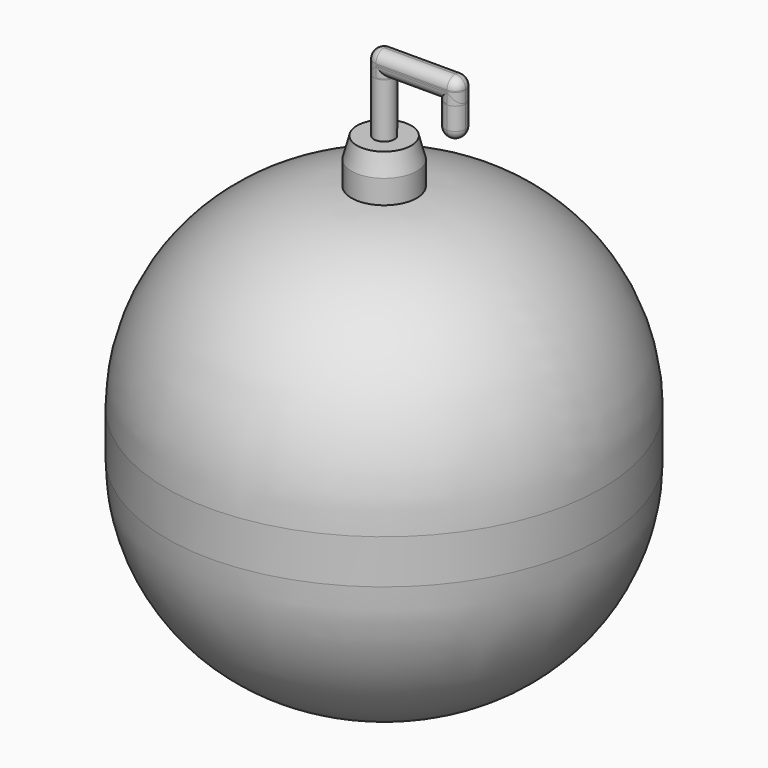
from build123d import *

# Parameters (mm, degrees)
F0_R          = 50
F0_R_2        = 7.5
F1_DEPTH      = 50
F0_R_3        = 2.3544117125
F3_DEPTH      = 50.038
F4_DEPTH      = 50.038
F5_DEPTH      = 10.16
F6_DEPTH      = 25.4
F8_DEPTH      = 2.54
F9_DEPTH      = 10.16
F10_SIZE2     = 4.7397045256
F10_SIZE      = 1.27
F11_R         = 2.286
F12_R         = 2.286
F13_DEPTH     = 2.54
F14_T4_DEPTH  = 27.7630922857
F14_S5_R      = 2.3587376624
F14_T6_DEPTH  = 15
F14_S7_R      = 2.3544117125
F14_T8_DEPTH  = 15
F14_T12_DEPTH = 27.7630922857
F14_S13_R     = 2.3587376624
F14_T14_DEPTH = 15
F14_S15_R     = 2.3544117125
F14_T16_DEPTH = 15


# Not quite as in the source:
# - a fillet or chamfer that OpenCascade refuses, or shapes differently, is made with other operations: its cross-section is extruded or revolved along the edge and cut away or added


with BuildPart() as f1:
    # F0 (on Top) → F1 (new body, symmetric)
    with BuildSketch(Plane.XY):
        Circle(F0_R)
        Circle(F0_R_2, mode=Mode.SUBTRACT)
    extrude(amount=F1_DEPTH, both=True)

    # F2: fillet of radius 45 on 3 edges, made by hand

    # F2_s1 → F2_t2 (revolve, cut)
    with BuildSketch(Plane.XZ):
        with BuildLine():
            ThreePointArc((50, 5.069498111), (37.6917420766, 35.9927903031), (7.5, 50))
            Line((7.5, 50), (50, 50))
            Line((50, 50), (50, 5.069498111))
        make_face()
    revolve(axis=Axis((0, 0, 50), (0, 0, 1)), mode=Mode.SUBTRACT)

    # F2_s3 → F2_t4 (revolve, cut)
    with BuildSketch(Plane.XZ):
        with BuildLine():
            ThreePointArc((50, -5.069498111), (37.6917420766, -35.9927903031), (7.5, -50))
            Line((7.5, -50), (50, -50))
            Line((50, -50), (50, -5.069498111))
        make_face()
    revolve(axis=Axis((0, 0, -50), (0, 0, 1)), mode=Mode.SUBTRACT)


with BuildPart() as f3:
    # F0 (on Top) → F3 (new body, symmetric)
    with BuildSketch(Plane.XY):
        Circle(F0_R_2)
        Circle(F0_R_3, mode=Mode.SUBTRACT)
    extrude(amount=F3_DEPTH, both=True)

    # F5 (add): a face of the model
    f5_faces = [f3.faces().sort_by_distance(p)[0] for p in [
        (-7.2878679656, 0, 50.038),
    ]]


with BuildPart() as f4:
    # F0 (on Top) → F4 (new body, symmetric)
    with BuildSketch(Plane.XY):
        Circle(F0_R_3)
    extrude(amount=F4_DEPTH, both=True)


with BuildPart() as f3_1:
    add(f3.part)

    add(f4.part)  # F5 merges F4
    extrude(f5_faces, amount=F5_DEPTH)

    # F6 (add): a face of the model
    f6_faces = [f3_1.faces().sort_by_distance(p)[0] for p in [
        (0, 0, 50.038),
    ]]
    extrude(f6_faces, amount=F6_DEPTH)

    # F7 (on face) → F8 (join)
    with BuildSketch(Plane.XY.offset(75.438)):
        with BuildLine():
            ThreePointArc((16.3282631107, -2.3587375796), (13.9701503516, 0), (16.3282631107, 2.3587375796))
            Line((16.3282631107, 2.3587375796), (0, 2.3544117125))
            ThreePointArc((0, 2.3544117125), (1.6648204876, 1.6648204876), (2.3544117125, 0))
            ThreePointArc((2.3544117125, 0), (1.6648204876, -1.6648204876), (0, -2.3544117125))
            Line((0, -2.3544117125), (16.3282631107, -2.3587375796))
        make_face()
        with BuildLine():
            Line((0, -2.3544117125), (0, 2.3544117125))
            ThreePointArc((0, 2.3544117125), (-2.3544117125, 0), (0, -2.3544117125))
        make_face()
        with BuildLine():
            ThreePointArc((2.3544117125, 0), (1.6648204876, 1.6648204876), (0, 2.3544117125))
            Line((0, 2.3544117125), (0, -2.3544117125))
            ThreePointArc((0, -2.3544117125), (1.6648204876, -1.6648204876), (2.3544117125, 0))
        make_face()
        with BuildLine():
            ThreePointArc((16.3282631107, -2.3587375796), (17.9965464588, -1.6681003182), (18.6876256764, 0))
            ThreePointArc((18.6876256764, 0), (17.9965464588, 1.6681003182), (16.3282631107, 2.3587375796))
            Line((16.3282631107, 2.3587375796), (16.3282631107, -2.3587375796))
        make_face()
        with BuildLine():
            Line((16.3282631107, -2.3587375796), (16.3282631107, 2.3587375796))
            ThreePointArc((16.3282631107, 2.3587375796), (13.9701503516, 0), (16.3282631107, -2.3587375796))
        make_face()
    extrude(amount=F8_DEPTH)

    # F7 (on face) → F9 (join)
    with BuildSketch(Plane.XY.offset(75.438)):
        with BuildLine():
            Line((16.3282631107, -2.3587375796), (16.3282631107, 2.3587375796))
            ThreePointArc((16.3282631107, 2.3587375796), (13.9701503516, 0), (16.3282631107, -2.3587375796))
        make_face()
        with BuildLine():
            ThreePointArc((16.3282631107, -2.3587375796), (17.9965464588, -1.6681003182), (18.6876256764, 0))
            ThreePointArc((18.6876256764, 0), (17.9965464588, 1.6681003182), (16.3282631107, 2.3587375796))
            Line((16.3282631107, 2.3587375796), (16.3282631107, -2.3587375796))
        make_face()
    extrude(amount=-F9_DEPTH)

    # F10
    f10_edges = [f3_1.edges().sort_by_distance(p)[0] for p in [
        (-7.5, 0, 60.198),
    ]]
    f10_side = f3_1.faces().sort_by_distance((-7.287868, 0, 60.198))[0]
    chamfer(f10_edges, length=F10_SIZE, length2=F10_SIZE2, reference=f10_side)

    # F11
    f11_edges = [f3_1.edges().sort_by_distance(p)[0] for p in [
        (8.164132, 2.356575, 77.978),
        (-2.354412, 0, 77.978),
        (8.164132, -2.356575, 77.978),
        (18.687626, 0, 77.978),
    ]]
    fillet(f11_edges, radius=F11_R)

    # F12
    f12_edges = [f3_1.edges().sort_by_distance(p)[0] for p in [
        (16.329513, 2.358738, 65.278),
    ]]
    fillet(f12_edges, radius=F12_R)

    # F7 (on face) → F13 (join)
    with BuildSketch(Plane.XY.offset(75.438)):
        with BuildLine():
            ThreePointArc((16.3282631107, -2.3587375796), (13.9701503516, 0), (16.3282631107, 2.3587375796))
            Line((16.3282631107, 2.3587375796), (0, 2.3544117125))
            ThreePointArc((0, 2.3544117125), (1.6648204876, 1.6648204876), (2.3544117125, 0))
            ThreePointArc((2.3544117125, 0), (1.6648204876, -1.6648204876), (0, -2.3544117125))
            Line((0, -2.3544117125), (16.3282631107, -2.3587375796))
        make_face()
    extrude(amount=-F13_DEPTH)

    # F14: fillet of radius 2.286 on 2 edges, made by hand


with BuildPart() as f14_tool2:
    # F14_s3 → F14_t4 (new body)
    with BuildSketch(Plane(origin=(22.0463009682, 0.005840754, 0), x_dir=(0, 0, 1), z_dir=(-0.9999999649, -0.0002649312, 0))):
        with BuildLine():
            ThreePointArc((75.1849656854, 2.3548116299), (73.5675538982, 1.6848577317), (72.8976, 0.0674459445))
            Line((72.8976, 0.0674459445), (72.6688634315, 0.0674459445))
            ThreePointArc((72.6688634315, 0.0674459445), (72.6692634315, 1.2109287872), (72.6692634315, 2.3544116299))
            Line((72.6692634315, 2.3544116299), (72.898, 2.5831481984))
            ThreePointArc((72.898, 2.5831481984), (74.0414828427, 2.5831481984), (75.1849656854, 2.5835481984))
            Line((75.1849656854, 2.5835481984), (75.1849656854, 2.3548116299))
        make_face()
    extrude(amount=F14_T4_DEPTH)

    # F14_s5 → F14_t6 (cut, symmetric)
    with BuildSketch(Plane.XY.offset(73.9)):
        with Locations((16.328888014, 0)):
            Circle(F14_S5_R)
    extrude(amount=F14_T6_DEPTH, both=True, mode=Mode.SUBTRACT)

    # F14_s7 → F14_t8 (cut, symmetric)
    with BuildSketch(Plane.XY.offset(73.9)):
        Circle(F14_S7_R)
    extrude(amount=F14_T8_DEPTH, both=True, mode=Mode.SUBTRACT)


with BuildPart() as f3_2:
    add(f3_1.part)

    # F14_t1: cut F14_tool2
    add(f14_tool2.part, mode=Mode.SUBTRACT)


with BuildPart() as f14_tool10:
    # F14_s11 → F14_t12 (new body)
    with BuildSketch(Plane(origin=(-5.7167903432, 0.0015145564, 0), x_dir=(0, 0, 1), z_dir=(0.9999999649, -0.0002649312, 0))):
        with BuildLine():
            ThreePointArc((72.8976, 0.0674459445), (73.5675538982, 1.6848577317), (75.1849656854, 2.3548116299))
            Line((75.1849656854, 2.3548116299), (75.1849656854, 2.5835481984))
            ThreePointArc((75.1849656854, 2.5835481984), (74.0414828427, 2.5831481984), (72.898, 2.5831481984))
            Line((72.898, 2.5831481984), (72.6692634315, 2.3544116299))
            ThreePointArc((72.6692634315, 2.3544116299), (72.6692634315, 1.2109287872), (72.6688634315, 0.0674459445))
            Line((72.6688634315, 0.0674459445), (72.8976, 0.0674459445))
        make_face()
    extrude(amount=F14_T12_DEPTH)

    # F14_s13 → F14_t14 (cut, symmetric)
    with BuildSketch(Plane.XY.offset(73.9)):
        with Locations((16.328888014, 0)):
            Circle(F14_S13_R)
    extrude(amount=F14_T14_DEPTH, both=True, mode=Mode.SUBTRACT)

    # F14_s15 → F14_t16 (cut, symmetric)
    with BuildSketch(Plane.XY.offset(73.9)):
        Circle(F14_S15_R)
    extrude(amount=F14_T16_DEPTH, both=True, mode=Mode.SUBTRACT)


with BuildPart() as f3_3:
    add(f3_2.part)

    # F14_t9: cut F14_tool10
    add(f14_tool10.part, mode=Mode.SUBTRACT)


solid = Compound([f1.part, f3_3.part])
